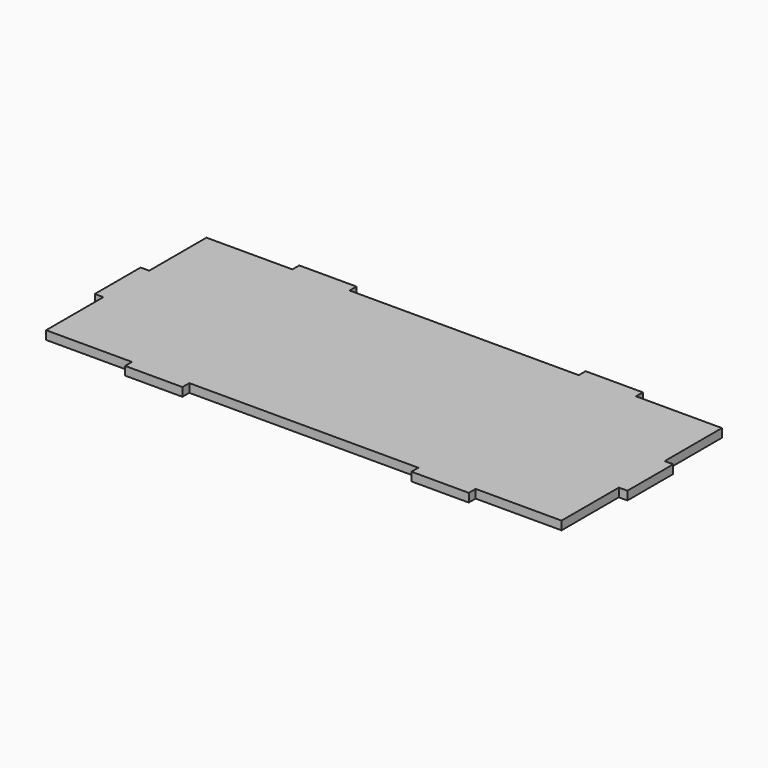
from build123d import *

# Parameters (mm, degrees)
F2_DEPTH = 3


# Not quite as in the source:
# - a feature names something its author has since deleted; it is built from what else it names


with BuildPart() as f2:
    # F1 (on Top) → F2 (new body)
    with BuildSketch(Plane.XY):
        Polygon((90, 10), (90, 35), (60, 35), (60, 38), (40, 38), (40, 35), (-40, 35), (-40, 38), (-60, 38), (-60, 35), (-90, 35), (-90, 10), (-93, 10), (-93, -10), (-90, -10), (-90, -35), (-60, -35), (-60, -38), (-40, -38), (-40, -35), (40, -35), (40, -38), (60, -38), (60, -35), (90, -35), (90, -10), (93, -10), (93, 10), align=None)
    extrude(amount=F2_DEPTH)


solid = f2.part
